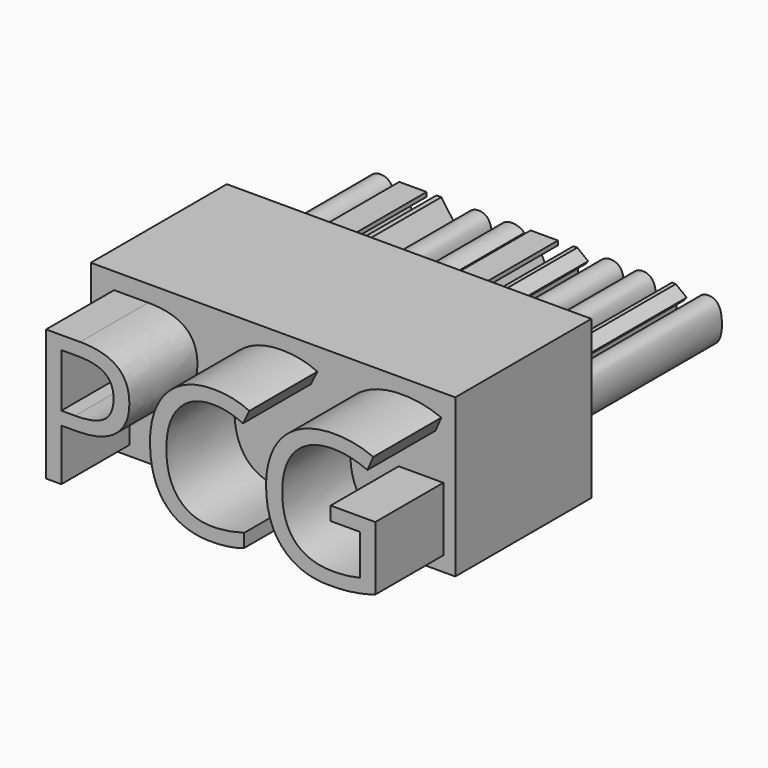
from build123d import *

# Parameters (mm, degrees)
F0_W         = 108.861528337
F0_H         = 47.1026599407
F1_DEPTH     = 50.8
F2_TEXT_SIZE = 54.9386574352
F3_DEPTH     = 25.4
F4_TEXT_SIZE = 17.1552412212
F5_DEPTH     = 50.8


# Not quite as in the source:
# - Text() gives the source's letters only with a copy of the font that has no kerning and outlines rounded to 1/6400 em; it was checked with that copy


with BuildPart() as f1:
    # F0 (on Front) → F1 (new body)
    with BuildSketch(Plane.XZ):
        with Locations((54.4307641685, 23.5513299704)):
            Rectangle(F0_W, F0_H)
    extrude(amount=F1_DEPTH)

    # F2 (on face) → F3 (join)
    with BuildSketch(Plane.XZ.offset(50.8)):
        with Locations((1.5852155296, 2.9379563363)):
            Text('PCG', F2_TEXT_SIZE, font='Open Sans', text_align=(TextAlign.LEFT, TextAlign.BOTTOM))
    extrude(amount=F3_DEPTH)

    # F4 (on face) → F5 (join)
    with BuildSketch(Plane(origin=(0, 0, 0), x_dir=(-1, 0, 0), z_dir=(0, 1, 0))):
        with Locations((-108.0807001999, 18.3433070779)):
            Text('01091720479', F4_TEXT_SIZE, font='Open Sans', text_align=(TextAlign.LEFT, TextAlign.BOTTOM))
    extrude(amount=F5_DEPTH)


solid = f1.part
